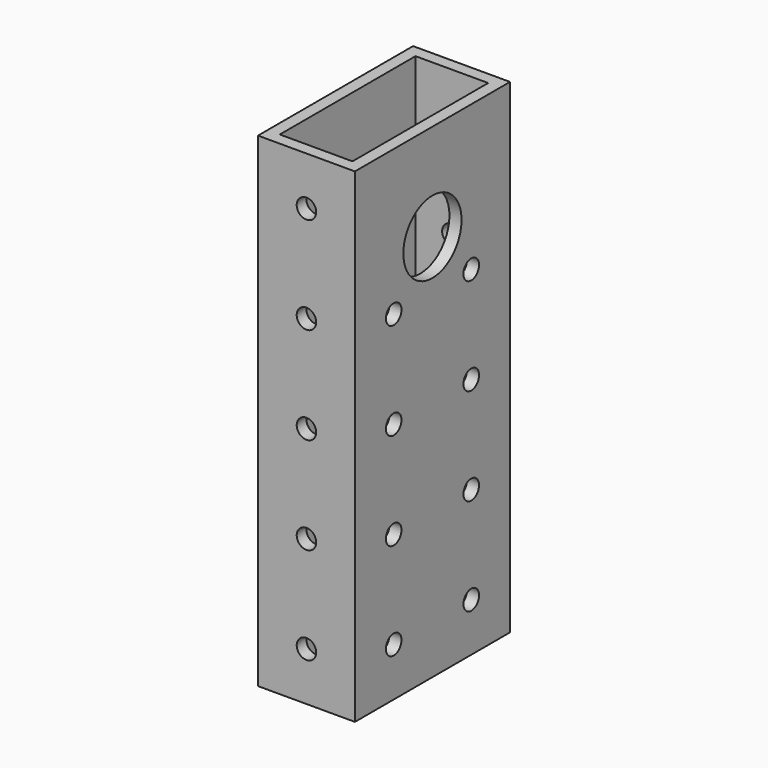
from build123d import *

# Parameters (mm, degrees)
F0_W     = 25.4
F0_H     = 50.8
F1_DEPTH = 127
F2_W     = 19.05
F2_H     = 44.45
F3_DEPTH = 127
F5_D     = 19.05
F6_D     = 5.1054
F8_D     = 5.1054


# Not quite as in the source:
# - a feature names something its author has since deleted; it is built from what else it names


with BuildPart() as f1:
    # F0 (on Top) → F1 (new body)
    with BuildSketch(Plane.XY):
        with Locations((-1.7230832018, 6.3088932174)):
            Rectangle(F0_W, F0_H)
    extrude(amount=F1_DEPTH)

    # F2 (on face) → F3 (cut)
    with BuildSketch(Plane.XY.offset(127)):
        with Locations((-1.7230832018, 6.3088932174)):
            Rectangle(F2_W, F2_H)
    extrude(amount=-F3_DEPTH, mode=Mode.SUBTRACT)

    # F5 (through all)
    with Locations(Plane.YZ.offset(10.9769167982)):
        with Locations((6.3088932174, 101.6)):
            Hole(F5_D / 2)

    # F6 (through all)
    with Locations(Plane.YZ.offset(10.9769167982)):
        with Locations((-6.3911067826, 63.5), (-6.3911067826, 88.9), (-6.3911067826, 38.1), (-6.3911067826, 12.7), (19.0088932174, 38.1), (19.0088932174, 12.7), (19.0088932174, 63.5), (19.0088932174, 88.9)):
            Hole(F6_D / 2)

    # F8 (through all)
    with Locations(Plane(origin=(0, 31.7088932174, 0), x_dir=(-1, 0, 0), z_dir=(0, 1, 0))):
        with Locations((1.7230832018, 88.9), (1.7230832018, 63.5), (1.7230832018, 114.3), (1.7230832018, 12.7), (1.7230832018, 38.1)):
            Hole(F8_D / 2)


solid = f1.part
